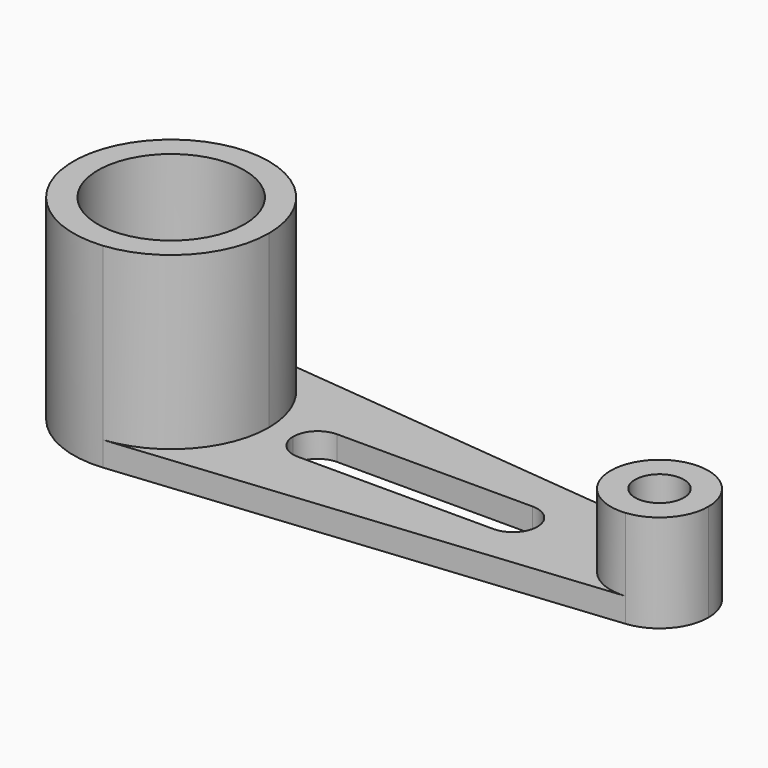
from build123d import *

# Parameters (mm, degrees)
F1_DEPTH = 6.35
F2_DEPTH = 25.4
F0_R     = 19.05
F3_DEPTH = 50.8


# Not quite as in the source:
# - a length typed as a fraction of an inch, garbled in the dataset ("3 / 203.2 mm" for 3/8 in), is restored


with BuildPart() as f1:
    # F0 (on Top) → F1 (new body)
    with BuildSketch(Plane.XY):
        with BuildLine():
            ThreePointArc((2.54, 25.2726809025), (18.8371441572, 17.0388379885), (25.4, 0))
            Line((25.4, 0), (31.75, 0))
            ThreePointArc((31.75, 0), (33.6098719395, 4.4901280605), (38.1, 6.35))
            Line((38.1, 6.35), (88.9, 6.35))
            ThreePointArc((88.9, 6.35), (93.3901280605, 4.4901280605), (95.25, 0))
            Line((95.25, 0), (114.3, 0))
            ThreePointArc((114.3, 0), (118.4805810057, 9.4185720786), (128.27, 12.6363404513))
            Line((128.27, 12.6363404513), (2.54, 25.2726809025))
        make_face()
        with BuildLine():
            Line((31.75, 0), (25.4, 0))
            ThreePointArc((25.4, 0), (18.8371441572, -17.0388379885), (2.54, -25.2726809025))
            Line((2.54, -25.2726809025), (128.27, -12.6363404513))
            ThreePointArc((128.27, -12.6363404513), (118.4805810057, -9.4185720786), (114.3, 0))
            Line((114.3, 0), (95.25, 0))
            ThreePointArc((95.25, 0), (93.3901280605, -4.4901280605), (88.9, -6.35))
            Line((88.9, -6.35), (38.1, -6.35))
            ThreePointArc((38.1, -6.35), (33.6098719395, -4.4901280605), (31.75, 0))
        make_face()
    extrude(amount=F1_DEPTH)

    # F0 (on Top) → F2 (join)
    with BuildSketch(Plane.XY):
        with BuildLine():
            ThreePointArc((139.7, 0), (136.4185720786, 8.5194189943), (128.27, 12.6363404513))
            ThreePointArc((128.27, 12.6363404513), (118.4805810057, 9.4185720786), (114.3, 0))
            ThreePointArc((114.3, 0), (118.4805810057, -9.4185720786), (128.27, -12.6363404513))
            ThreePointArc((128.27, -12.6363404513), (136.4185720786, -8.5194189943), (139.7, 0))
        make_face()
        with BuildLine():
            ThreePointArc((133.35, 0), (127, -6.35), (120.65, 0))
            ThreePointArc((120.65, 0), (127, 6.35), (133.35, 0))
        make_face(mode=Mode.SUBTRACT)
    extrude(amount=F2_DEPTH)

    # F0 (on Top) → F3 (join)
    with BuildSketch(Plane.XY):
        with BuildLine():
            ThreePointArc((2.54, -25.2726809025), (18.8371441572, -17.0388379885), (25.4, 0))
            ThreePointArc((25.4, 0), (18.8371441572, 17.0388379885), (2.54, 25.2726809025))
            ThreePointArc((2.54, 25.2726809025), (-25.4, 0), (2.54, -25.2726809025))
        make_face()
        Circle(F0_R, mode=Mode.SUBTRACT)
    extrude(amount=F3_DEPTH)


solid = f1.part
